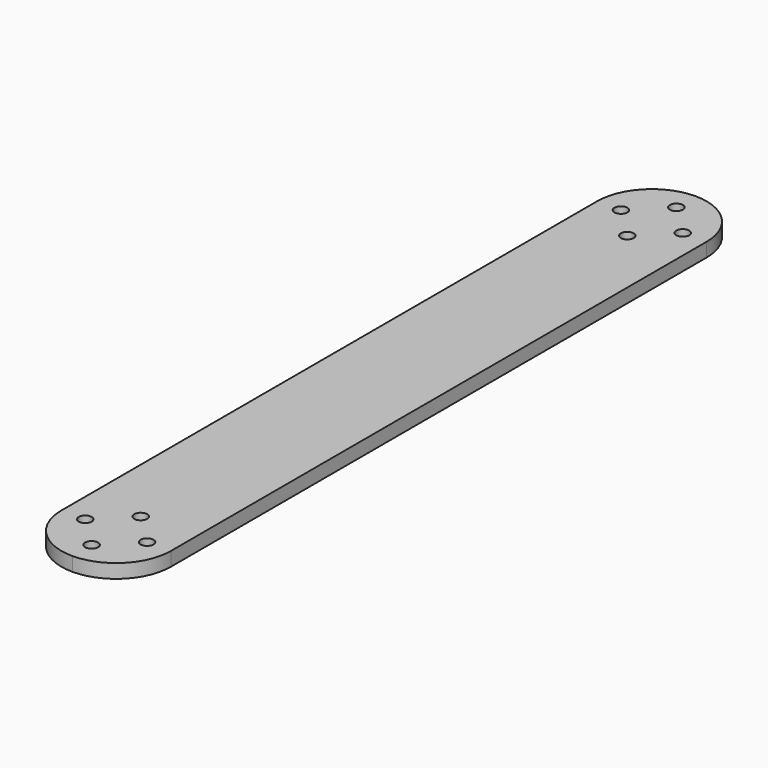
from build123d import *

# Parameters (mm, degrees)
F0_R     = 1.4732
F1_DEPTH = 3.175


# Not quite as in the source:
# - a length typed as a fraction of an inch, garbled in the dataset ("3 / 203.2 mm" for 3/8 in), is restored


with BuildPart() as f1:
    # F0 (on Top) → F1 (new body)
    with BuildSketch(Plane.XY):
        with BuildLine():
            Line((12.5, -76.4), (12.5, 76.4))
            ThreePointArc((12.5, 76.4), (8.8388347648, 85.2388347648), (0, 88.9))
            ThreePointArc((0, 88.9), (-8.8388347648, 85.2388347648), (-12.5, 76.4))
            Line((-12.5, 76.4), (-12.5, -76.4))
            ThreePointArc((-12.5, -76.4), (-8.8388347648, -85.2388347648), (0, -88.9))
            ThreePointArc((0, -88.9), (8.8388347648, -85.2388347648), (12.5, -76.4))
        make_face()
        with Locations((-7.0527177304, -76.4)):
            Circle(F0_R, mode=Mode.SUBTRACT)
        with Locations((0, -83.4)):
            Circle(F0_R, mode=Mode.SUBTRACT)
        with Locations((0, -69.4)):
            Circle(F0_R, mode=Mode.SUBTRACT)
        with Locations((7.0527177304, -76.4)):
            Circle(F0_R, mode=Mode.SUBTRACT)
        with Locations((-7.0527177304, 76.4)):
            Circle(F0_R, mode=Mode.SUBTRACT)
        with Locations((0, 69.4)):
            Circle(F0_R, mode=Mode.SUBTRACT)
        with Locations((0, 83.4)):
            Circle(F0_R, mode=Mode.SUBTRACT)
        with Locations((7.0527177304, 76.4)):
            Circle(F0_R, mode=Mode.SUBTRACT)
    extrude(amount=F1_DEPTH)


solid = f1.part
